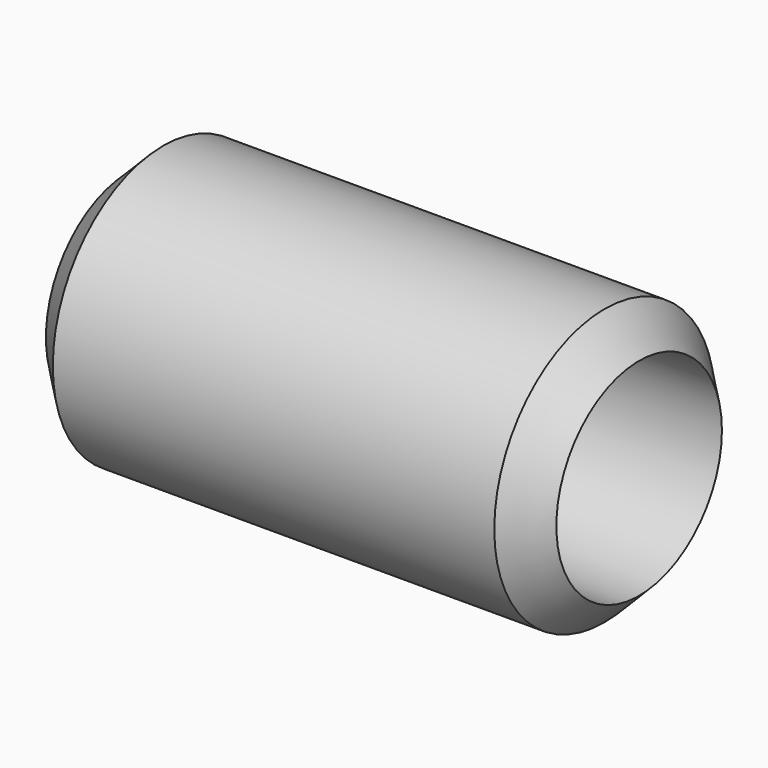
from build123d import *

# Parameters (mm, degrees)
F0_R     = 12.7
F0_R_2   = 9.525
F1_DEPTH = 50.8


# Not quite as in the source:
# - a fillet or chamfer that OpenCascade refuses, or shapes differently, is made with other operations: its cross-section is extruded or revolved along the edge and cut away or added


with BuildPart() as f1:
    # F0 (on Right) → F1 (new body)
    with BuildSketch(Plane.YZ):
        Circle(F0_R)
        Circle(F0_R_2, mode=Mode.SUBTRACT)
    extrude(amount=F1_DEPTH)

    # F2: chamfer of 5.08 on 3 edges, made by hand

    # F2_s1 → F2_t2 (revolve, cut)
    with BuildSketch(Plane.XY):
        Polygon((45.72, 12.7), (50.8, 7.62), (50.8, 12.7), align=None)
    revolve(axis=Axis((50.8, 0, 0), (1, 0, 0)), mode=Mode.SUBTRACT)

    # F2_s3 → F2_t4 (revolve, cut)
    with BuildSketch(Plane.XY):
        Polygon((5.08, 12.7), (0, 7.62), (0, 12.7), align=None)
    revolve(axis=Axis((0, 0, 0), (1, 0, 0)), mode=Mode.SUBTRACT)


solid = f1.part
